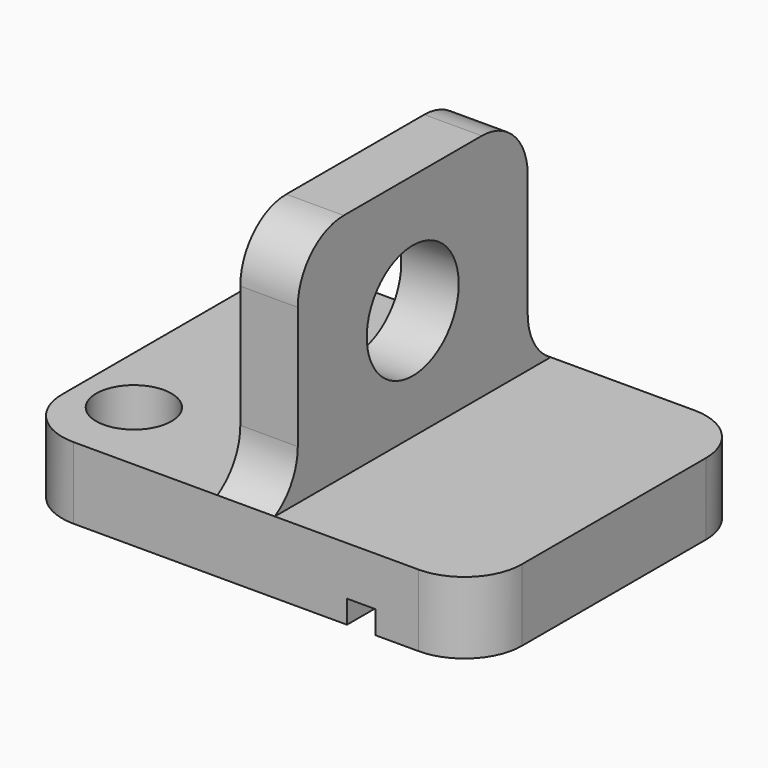
from build123d import *

# Parameters (mm, degrees)
F0_W        = 40
F0_H        = 30
F1_DEPTH    = 6.25
F2_R        = 5
F3_W        = 5
F3_H        = 25
F4_DEPTH    = 20
F5_T1_DEPTH = 5
F5_T3_DEPTH = 5
F5_T5_DEPTH = 30
F5_T7_DEPTH = 30
F7_R        = 5
F8_DEPTH    = 5
F6_R        = 3.275
F9_DEPTH    = 25
F10_W       = 2.5
F10_H       = 30
F11_DEPTH   = 2


# Not quite as in the source:
# - a fillet or chamfer that OpenCascade refuses, or shapes differently, is made with other operations: its cross-section is extruded or revolved along the edge and cut away or added


with BuildPart() as f1:
    # F0 (on Top) → F1 (new body)
    with BuildSketch(Plane.XY):
        with Locations((1.2747282162, -9.7165126197)):
            Rectangle(F0_W, F0_H)
    extrude(amount=F1_DEPTH)

    # F2
    f2_edges = [f1.edges().sort_by_distance(p)[0] for p in [
        (-18.725272, -24.716513, 3.125),
        (21.274728, -24.716513, 3.125),
        (21.274728, 5.283487, 3.125),
        (-18.725272, 5.283487, 3.125),
    ]]
    fillet(f2_edges, radius=F2_R)

    # F3 (on face) → F4 (join)
    with BuildSketch(Plane.XY.offset(6.25)):
        with Locations((1.2747282162, -9.7165126197)):
            Rectangle(F3_W, F3_H)
    extrude(amount=F4_DEPTH)

    # F5: fillet of radius 5 on 4 edges, made by hand

    # F5_s2 → F5_t1 (join)
    with BuildSketch(Plane.YZ.offset(-1.2252717838)):
        with BuildLine():
            ThreePointArc((5.2834873803, 6.25), (3.4533603614, 8.0801270189), (2.7834873803, 10.5801270189))
            Line((2.7834873803, 10.5801270189), (2.7834873803, 6.25))
            Line((2.7834873803, 6.25), (5.2834873803, 6.25))
        make_face()
    extrude(amount=F5_T1_DEPTH)

    # F5_s4 → F5_t3 (join)
    with BuildSketch(Plane.YZ.offset(-1.2252717838)):
        with BuildLine():
            ThreePointArc((-24.7165126197, 6.25), (-22.8863856008, 8.0801270189), (-22.2165126197, 10.5801270189))
            Line((-22.2165126197, 10.5801270189), (-22.2165126197, 6.25))
            Line((-22.2165126197, 6.25), (-24.7165126197, 6.25))
        make_face()
    extrude(amount=F5_T3_DEPTH)

    # F5_s6 → F5_t5 (cut)
    with BuildSketch(Plane.YZ.offset(-13.7252717838)):
        with BuildLine():
            ThreePointArc((2.7834873803, 21.25), (1.3190212862, 24.7855339059), (-2.2165126197, 26.25))
            Line((-2.2165126197, 26.25), (2.7834873803, 26.25))
            Line((2.7834873803, 26.25), (2.7834873803, 21.25))
        make_face()
    extrude(amount=F5_T5_DEPTH, mode=Mode.SUBTRACT)

    # F5_s8 → F5_t7 (cut)
    with BuildSketch(Plane.YZ.offset(-13.7252717838)):
        with BuildLine():
            ThreePointArc((-22.2165126197, 21.25), (-20.7520465256, 24.7855339059), (-17.2165126197, 26.25))
            Line((-17.2165126197, 26.25), (-22.2165126197, 26.25))
            Line((-22.2165126197, 26.25), (-22.2165126197, 21.25))
        make_face()
    extrude(amount=F5_T7_DEPTH, mode=Mode.SUBTRACT)

    # F7 (on face) → F8 (cut)
    with BuildSketch(Plane.YZ.offset(3.7747282162)):
        with Locations((-9.7165126197, 15.9150635095)):
            Circle(F7_R)
    extrude(amount=-F8_DEPTH, mode=Mode.SUBTRACT)

    # F6 (on face) → F9 (cut)
    with BuildSketch(Plane.XY.offset(6.25)):
        with Locations((-13.7252717838, -1.2665126197)):
            Circle(F6_R)
        with Locations((-13.7252717838, -18.1665126197)):
            Circle(F6_R)
    extrude(amount=-F9_DEPTH, mode=Mode.SUBTRACT)

    # F10 (on face) → F11 (cut)
    with BuildSketch(Plane(origin=(0, 0, 0), x_dir=(1, 0, 0), z_dir=(0, 0, -1))):
        with Locations((11.3062032312, 9.7165126197)):
            Rectangle(F10_W, F10_H)
    extrude(amount=-F11_DEPTH, mode=Mode.SUBTRACT)


solid = f1.part
